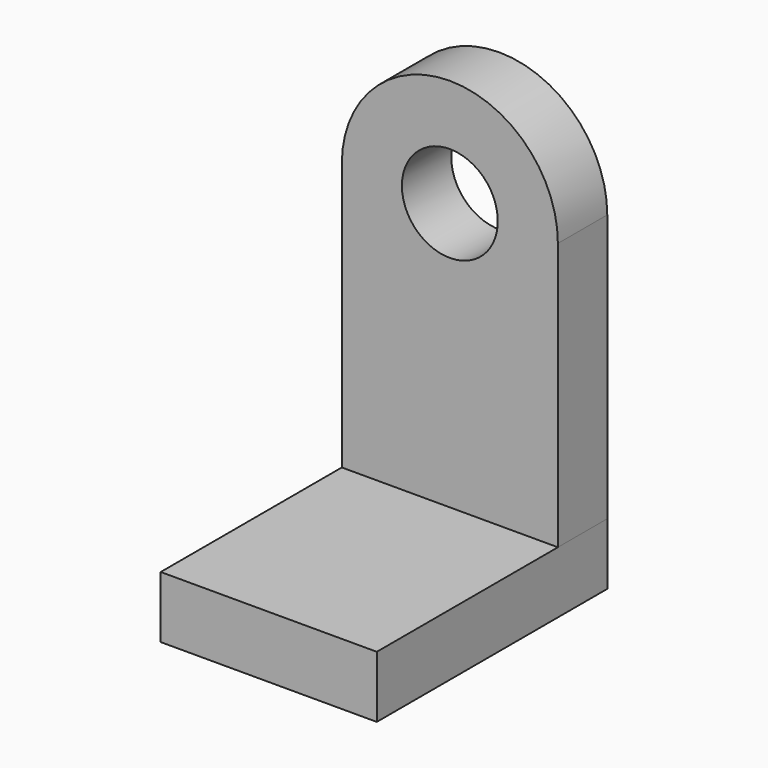
from build123d import *

# Parameters (mm, degrees)
F0_W          = 105
F0_H          = 30
F1_DEPTH      = 110
F1_DEPTH_BACK = 30
F2_DEPTH      = 30


# Not quite as in the source:
# - a feature of the source that left no trace in its solid (it failed there, or was rolled back) is left out


with BuildPart() as f1:
    # F0 (on Front) → F1 (new body, two sides)
    with BuildSketch(Plane.XZ) as f1_sk:
        with Locations((52.5, 15)):
            Rectangle(F0_W, F0_H)
    extrude(amount=F1_DEPTH)
    extrude(f1_sk.sketch, amount=-F1_DEPTH_BACK)


with BuildPart() as f2:
    # F0 (on Front) → F2 (new body)
    with BuildSketch(Plane.XZ):
        with BuildLine():
            Line((0, 160), (0, 30))
            Line((0, 30), (105, 30))
            Line((105, 30), (105, 160))
            Line((105, 160), (75.8, 160))
            ThreePointArc((75.8, 160), (52.5, 136.7), (29.2, 160))
            Line((29.2, 160), (0, 160))
        make_face()
        with BuildLine():
            ThreePointArc((105, 160), (52.5, 212.5), (0, 160))
            Line((0, 160), (29.2, 160))
            ThreePointArc((29.2, 160), (52.5, 183.3), (75.8, 160))
            Line((75.8, 160), (105, 160))
        make_face()
    extrude(amount=-F2_DEPTH)


solid = Compound([f1.part, f2.part])
